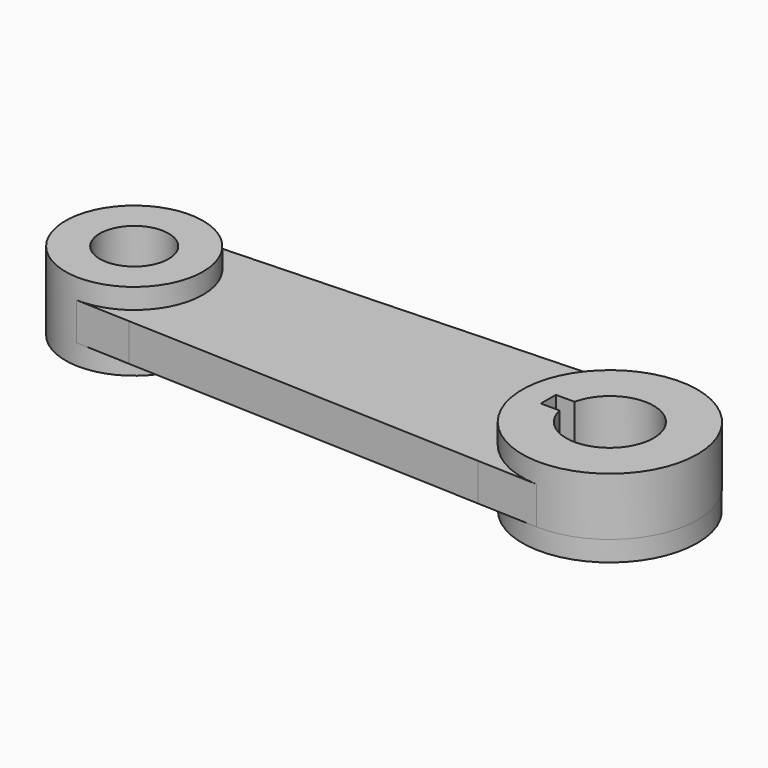
from build123d import *

# Parameters (mm, degrees)
F0_R     = 5.5
F1_DEPTH = 6
F4_DEPTH = 3.25
F2_R     = 13.9763796755
F5_DEPTH = 3.25
F3_R     = 5.5
F6_DEPTH = 3.25
F7_R     = 5.5
F8_DEPTH = 3.25


with BuildPart() as f1:
    # F0 (on Top) → F1 (new body)
    with BuildSketch(Plane.XY):
        with BuildLine():
            ThreePointArc((27.8112338211, -13.6084181209), (21, 0), (27.8112338211, 13.6084181209))
            Line((27.8112338211, 13.6084181209), (-29.7807062004, 11.3332788475))
            ThreePointArc((-29.7807062004, 11.3332788475), (-24, 0), (-29.7807062004, -11.3332788475))
            Line((-29.7807062004, -11.3332788475), (27.8112338211, -13.6084181209))
        make_face()
        with BuildLine():
            ThreePointArc((-29.7807062004, -11.3332788475), (-24, 0), (-29.7807062004, 11.3332788475))
            Line((-29.7807062004, 11.3332788475), (-38.4342105263, 10.9914267144))
            ThreePointArc((-38.4342105263, 10.9914267144), (-30.3768876366, 7.9302054131), (-27, 0))
            ThreePointArc((-27, 0), (-30.3768876366, -7.9302054131), (-38.4342105263, -10.9914267144))
            Line((-38.4342105263, -10.9914267144), (-29.7807062004, -11.3332788475))
        make_face()
        with BuildLine():
            ThreePointArc((-27, 0), (-30.3768876366, 7.9302054131), (-38.4342105263, 10.9914267144))
            ThreePointArc((-38.4342105263, 10.9914267144), (-49, 0), (-38.4342105263, -10.9914267144))
            ThreePointArc((-38.4342105263, -10.9914267144), (-30.3768876366, -7.9302054131), (-27, 0))
        make_face()
        with Locations((-38, 0)):
            Circle(F0_R, mode=Mode.SUBTRACT)
        with BuildLine():
            ThreePointArc((37.4473684211, -13.9890885456), (24, 0), (37.4473684211, 13.9890885456))
            Line((37.4473684211, 13.9890885456), (27.8112338211, 13.6084181209))
            ThreePointArc((27.8112338211, 13.6084181209), (21, 0), (27.8112338211, -13.6084181209))
            Line((27.8112338211, -13.6084181209), (37.4473684211, -13.9890885456))
        make_face()
        with BuildLine():
            ThreePointArc((37.4473684211, -13.9890885456), (47.702143008, -10.0929887076), (52, 0))
            ThreePointArc((52, 0), (47.702143008, 10.0929887076), (37.4473684211, 13.9890885456))
            ThreePointArc((37.4473684211, 13.9890885456), (24, 0), (37.4473684211, -13.9890885456))
        make_face()
        with BuildLine():
            ThreePointArc((31.1628594053, 1.5011690405), (44.9999998977, -0.0011968644), (31.1623464634, -1.4988309156))
            Line((31.1623464634, -1.4988309156), (28.1623464634, -1.4988309156))
            Line((28.1623464634, -1.4988309156), (28.1628594053, 1.5011690405))
            Line((28.1628594053, 1.5011690405), (31.1628594053, 1.5011690405))
        make_face(mode=Mode.SUBTRACT)
    extrude(amount=F1_DEPTH)

    # F3 (on face) → F4 (join)
    with BuildSketch(Plane.XY.offset(6)):
        with BuildLine():
            ThreePointArc((52, 0), (47.702143008, 10.0929887076), (37.4473684211, 13.9890885456))
            ThreePointArc((37.4473684211, 13.9890885456), (24, 0), (37.4473684211, -13.9890885456))
            ThreePointArc((37.4473684211, -13.9890885456), (47.702143008, -10.0929887076), (52, 0))
        make_face()
        with BuildLine():
            Line((31.1623464634, -1.4988309156), (28.1623464634, -1.4988309156))
            Line((28.1623464634, -1.4988309156), (28.1628594053, 1.5011690405))
            Line((28.1628594053, 1.5011690405), (31.1628594053, 1.5011690405))
            ThreePointArc((31.1628594053, 1.5011690405), (44.9999998977, -0.0011968644), (31.1623464634, -1.4988309156))
        make_face(mode=Mode.SUBTRACT)
    extrude(amount=F4_DEPTH)

    # F2 (on face) → F5 (join)
    with BuildSketch(Plane(origin=(0, 0, 0), x_dir=(1, 0, 0), z_dir=(0, 0, -1))):
        with Locations((38, 0)):
            Circle(F2_R)
        with BuildLine():
            Line((28.1623464634, 1.4988309156), (31.1623464634, 1.4988309156))
            ThreePointArc((31.1623464634, 1.4988309156), (44.9999998977, 0.0011968644), (31.1628594053, -1.5011690405))
            Line((31.1628594053, -1.5011690405), (28.1628594053, -1.5011690405))
            Line((28.1628594053, -1.5011690405), (28.1623464634, 1.4988309156))
        make_face(mode=Mode.SUBTRACT)
    extrude(amount=F5_DEPTH)

    # F3 (on face) → F6 (join)
    with BuildSketch(Plane.XY.offset(6)):
        with BuildLine():
            ThreePointArc((-38.4342105263, -10.9914267144), (-30.3768876366, -7.9302054131), (-27, 0))
            ThreePointArc((-27, 0), (-30.3768876366, 7.9302054131), (-38.4342105263, 10.9914267144))
            ThreePointArc((-38.4342105263, 10.9914267144), (-49, 0), (-38.4342105263, -10.9914267144))
        make_face()
        with Locations((-38, 0)):
            Circle(F3_R, mode=Mode.SUBTRACT)
    extrude(amount=F6_DEPTH)

    # F7 (on face) → F8 (join)
    with BuildSketch(Plane(origin=(0, 0, 0), x_dir=(1, 0, 0), z_dir=(0, 0, -1))):
        with BuildLine():
            ThreePointArc((-38.4342105263, -10.9914267144), (-30.3768876366, -7.9302054131), (-27, 0))
            ThreePointArc((-27, 0), (-30.3768876366, 7.9302054131), (-38.4342105263, 10.9914267144))
            ThreePointArc((-38.4342105263, 10.9914267144), (-49, 0), (-38.4342105263, -10.9914267144))
        make_face()
        with Locations((-38, 0)):
            Circle(F7_R, mode=Mode.SUBTRACT)
    extrude(amount=F8_DEPTH)


solid = f1.part
